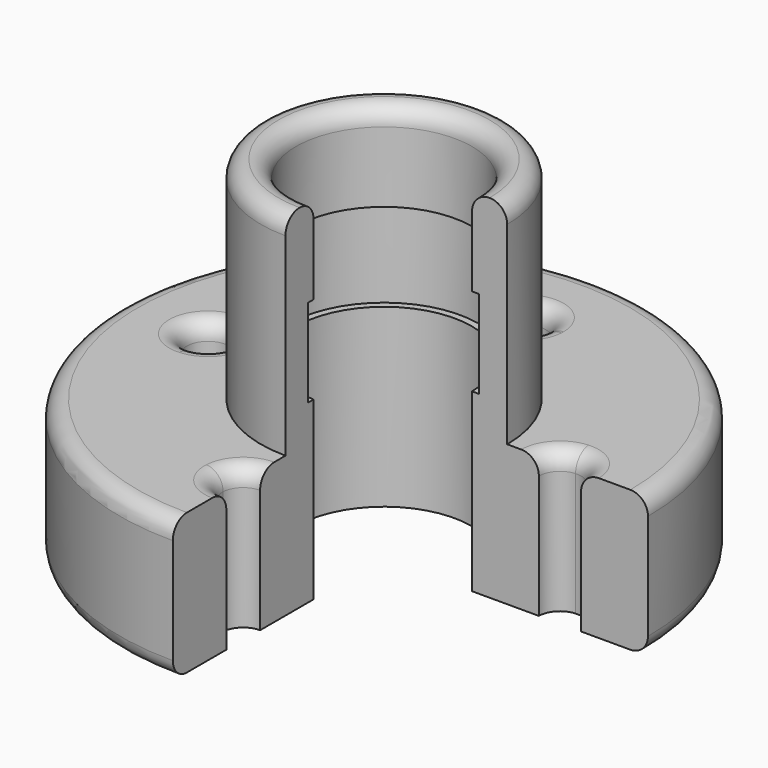
from build123d import *

# Parameters (mm, degrees)
F1_ANGLE = 270
F3_DEPTH = 1000
F4_R     = 4.99999


# Not quite as in the source:
# - a fillet or chamfer is up to 0.001 mm smaller than in the source, because OpenCascade refuses the exact size


with BuildPart() as f1:
    # F0 (on Front) → F1 (revolve)
    with BuildSketch(Plane.XZ):
        Polygon((25, 50), (25, 0), (35, 0), (75, 0), (75, 40), (35, 40), (35, 100), (25, 100), (25, 75), (27, 75), (27, 50), align=None)
    revolve(axis=Axis((0, 0, 36.062438041), (0, 0, 1)), revolution_arc=F1_ANGLE)

    # F2 (on Top) → F3 (cut)
    with BuildSketch(Plane.XY):
        with BuildLine():
            ThreePointArc((-44, 0), (-45.6319340664, 4.1133927602), (-49.64, 5.9891902625))
            ThreePointArc((-49.64, 5.9891902625), (-50, 0), (-49.64, -5.9891902625))
            ThreePointArc((-49.64, -5.9891902625), (-45.6319340664, -4.1133927602), (-44, 0))
        make_face()
        with BuildLine():
            ThreePointArc((-49.64, -5.9891902625), (-50, 0), (-49.64, 5.9891902625))
            ThreePointArc((-49.64, 5.9891902625), (-56, 0), (-49.64, -5.9891902625))
        make_face()
        with BuildLine():
            ThreePointArc((-5.9891902625, 49.64), (0, 44), (5.9891902625, 49.64))
            ThreePointArc((5.9891902625, 49.64), (0, 50), (-5.9891902625, 49.64))
        make_face()
        with BuildLine():
            ThreePointArc((-5.9891902625, 49.64), (0, 50), (5.9891902625, 49.64))
            ThreePointArc((5.9891902625, 49.64), (5.9972969567, 49.8199188722), (6, 50))
            ThreePointArc((6, 50), (-0.1800811278, 55.9972969567), (-5.9891902625, 49.64))
        make_face()
        with BuildLine():
            ThreePointArc((49.64, -5.9891902625), (49.9099188539, -3), (50, 0))
            ThreePointArc((50, 0), (49.9099188539, 3), (49.64, 5.9891902625))
            ThreePointArc((49.64, 5.9891902625), (44, 0), (49.64, -5.9891902625))
        make_face()
        with BuildLine():
            ThreePointArc((49.64, 5.9891902625), (49.9099188539, 3), (50, 0))
            ThreePointArc((50, 0), (49.9099188539, -3), (49.64, -5.9891902625))
            ThreePointArc((49.64, -5.9891902625), (54.1133927602, -4.3680659336), (56, 0))
            ThreePointArc((56, 0), (54.1133927602, 4.3680659336), (49.64, 5.9891902625))
        make_face()
        with BuildLine():
            ThreePointArc((-5.9891902625, -49.64), (0, -50), (5.9891902625, -49.64))
            ThreePointArc((5.9891902625, -49.64), (0, -44), (-5.9891902625, -49.64))
        make_face()
        with BuildLine():
            ThreePointArc((6, -50), (5.9972969567, -49.8199188722), (5.9891902625, -49.64))
            ThreePointArc((5.9891902625, -49.64), (0, -50), (-5.9891902625, -49.64))
            ThreePointArc((-5.9891902625, -49.64), (-0.1800811278, -55.9972969567), (6, -50))
        make_face()
    extrude(amount=F3_DEPTH, mode=Mode.SUBTRACT)

    # F4 (radius 5 in the source; OpenCascade refuses exactly that, so slightly less here)
    f4_edges = [f1.edges().sort_by_distance(p)[0] for p in [
        (-24.748737, 24.748737, 100),
        (-17.67767, 17.67767, 100),
        (-53.033009, 53.033009, 40),
        (-56, 0, 40),
        (-6, -50, 40),
        (50, 6, 40),
        (-5.98919, 50.36, 40),
        (-53.033009, 53.033009, 0),
    ]]
    fillet(f4_edges, radius=F4_R)


solid = f1.part
